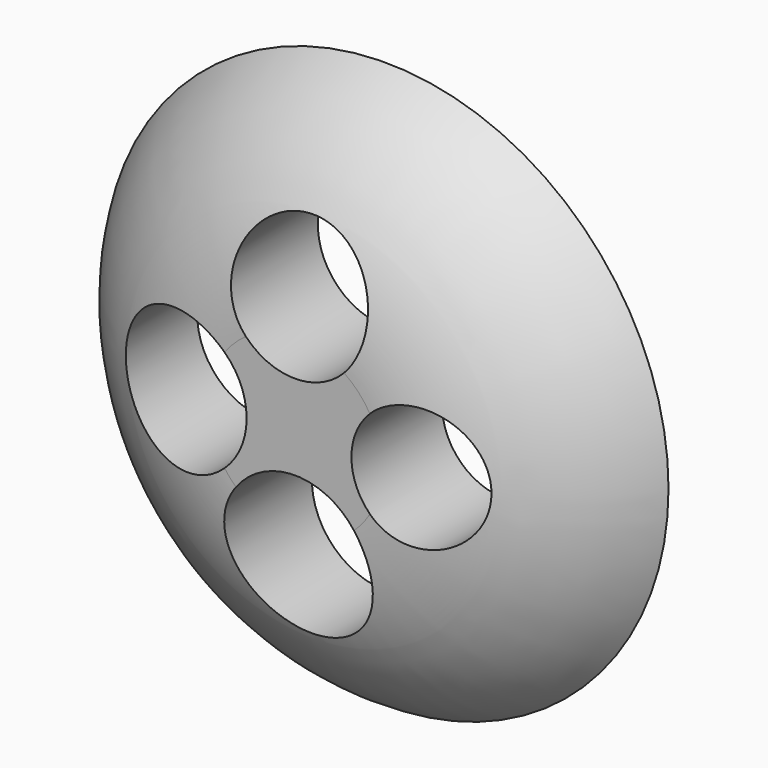
from build123d import *

# Parameters (mm, degrees)
F0_R     = 6.35
F0_R_2   = 1.6535683919
F0_R_3   = 1.5708348414
F0_R_4   = 1.3906858061
F0_R_5   = 1.5190356383
F1_DEPTH = 2.54


# Not quite as in the source:
# - a fillet or chamfer that OpenCascade refuses, or shapes differently, is made with other operations: its cross-section is extruded or revolved along the edge and cut away or added


with BuildPart() as f1:
    # F0 (on Front) → F1 (new body)
    with BuildSketch(Plane.XZ):
        Circle(F0_R)
        with Locations((0, -2.4252922231)):
            Circle(F0_R_2, mode=Mode.SUBTRACT)
        with Locations((-2.6562736366, 0)):
            Circle(F0_R_3, mode=Mode.SUBTRACT)
        with Locations((2.6562768198, 0)):
            Circle(F0_R_4, mode=Mode.SUBTRACT)
        with Locations((0, 2.6562763651)):
            Circle(F0_R_5, mode=Mode.SUBTRACT)
    extrude(amount=F1_DEPTH)

    # F2: fillet of radius 5.08 on 1 edges, made by hand

    # F2_s1 → F2_t2 (revolve, cut)
    with BuildSketch(Plane.XY):
        with BuildLine():
            ThreePointArc((6.35, 0), (4.4905909488, -1.8594090512), (1.9505909488, -2.54))
            Line((1.9505909488, -2.54), (6.35, -2.54))
            Line((6.35, -2.54), (6.35, 0))
        make_face()
    revolve(axis=Axis((0, -2.54, 0), (0, -1, 0)), mode=Mode.SUBTRACT)


solid = f1.part
